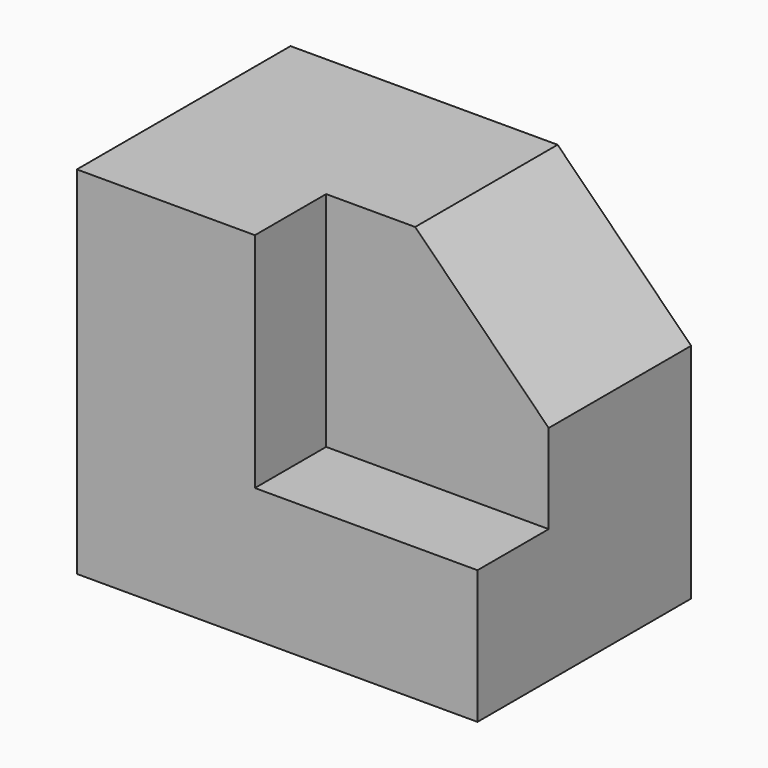
from build123d import *

# Parameters (mm, degrees)
F0_W     = 228.6
F0_H     = 152.4
F1_DEPTH = 203.2
F2_W     = 127
F2_H     = 50.8
F3_DEPTH = 127
F5_DEPTH = 101.6


# Not quite as in the source:
# - a feature names something its author has since deleted; it is built from what else it names


with BuildPart() as f1:
    # F0 (on Top) → F1 (new body)
    with BuildSketch(Plane.XY):
        with Locations((10.0263133645, -15.0303587328)):
            Rectangle(F0_W, F0_H)
    extrude(amount=F1_DEPTH)

    # F2 (on face) → F3 (cut)
    with BuildSketch(Plane.XY.offset(203.2)):
        with Locations((60.8263133645, -65.8303587328)):
            Rectangle(F2_W, F2_H)
    extrude(amount=-F3_DEPTH, mode=Mode.SUBTRACT)

    # F4 (on face) → F5 (cut)
    with BuildSketch(Plane.XZ.offset(40.4303587328)):
        Polygon((124.3263133645, 203.2), (48.1263133645, 203.2), (124.3263133645, 127), align=None)
    extrude(amount=-F5_DEPTH, mode=Mode.SUBTRACT)


solid = f1.part
